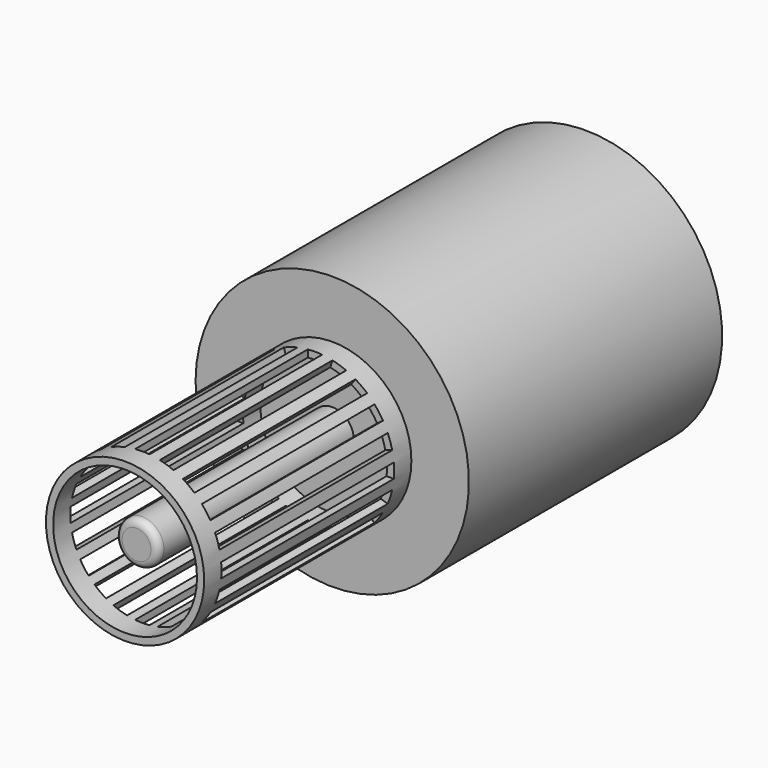
from build123d import *

# Parameters (mm, degrees)
F0_R            = 5.5
F0_R_2          = 5
F1_DEPTH        = 35
F2_W            = 18
F2_H            = 30
F3_DEPTH        = 25
F3_DEPTH_BACK   = 25
F4_R            = 7.5
F4_R_2          = 5.5
F4_R_3          = 5
F5_DEPTH        = 2
F6_W            = 15
F6_H            = 1
F7_DEPTH        = 10
F7_COPIES_COUNT = 20
F8_R            = 1.5
F9_DEPTH        = 19
F11_R           = 9.5
F11_R_2         = 9
F11_R_3         = 7.5
F12_DEPTH       = 2
F13_DEPTH       = 20
F14_R           = 0.5


# Not quite as in the source:
# - a pattern or mirror of a feature is missing from the dataset's text; its kind, count and spacing are read off the source's solid


with BuildPart() as f1:
    # F0 (on Front) → F1 (new body)
    with BuildSketch(Plane.XZ):
        Circle(F0_R)
        Circle(F0_R_2, mode=Mode.SUBTRACT)
    extrude(amount=F1_DEPTH)

    # F2 (on Top) → F3 (cut, two sides)
    with BuildSketch(Plane.XY) as f3_sk:
        Rectangle(F2_W, F2_H)
    extrude(amount=F3_DEPTH, mode=Mode.SUBTRACT)
    extrude(f3_sk.sketch, amount=-F3_DEPTH_BACK, mode=Mode.SUBTRACT)

    # F4 (on face) → F5 (join)
    with BuildSketch(Plane(origin=(0, -15, 0), x_dir=(-1, 0, 0), z_dir=(0, 1, 0))):
        Circle(F4_R)
        Circle(F4_R_2, mode=Mode.SUBTRACT)
        Circle(F4_R_3)
    extrude(amount=-F5_DEPTH)

    # F6 (on Right) → F7 (cut)
    with BuildSketch(Plane.YZ):
        with Locations((-26, 0)):
            Rectangle(F6_W, F6_H)
    f7 = extrude(amount=-F7_DEPTH, mode=Mode.SUBTRACT)

    # F7_copies: F7 ×20 about axis
    f7_copies_axis = Axis((0, 0, 0), (0, 1, 0))
    for i in range(1, F7_COPIES_COUNT):
        add(f7.rotate(f7_copies_axis, i * 360 / F7_COPIES_COUNT), mode=Mode.SUBTRACT)

    # F8 (on face) → F9 (join)
    with BuildSketch(Plane(origin=(0, -15, 0), x_dir=(-1, 0, 0), z_dir=(0, 1, 0))):
        Circle(F8_R)
    extrude(amount=-F9_DEPTH)

    # F11 (on face) → F12 (join)
    with BuildSketch(Plane(origin=(0, -15, 0), x_dir=(-1, 0, 0), z_dir=(0, 1, 0))):
        Circle(F11_R)
        Circle(F11_R_2, mode=Mode.SUBTRACT)
        Circle(F11_R_2)
        Circle(F11_R_3, mode=Mode.SUBTRACT)
    extrude(amount=-F12_DEPTH)

    # F11 (on face) → F13 (join)
    with BuildSketch(Plane(origin=(0, -15, 0), x_dir=(-1, 0, 0), z_dir=(0, 1, 0))):
        Circle(F11_R)
        Circle(F11_R_2, mode=Mode.SUBTRACT)
    extrude(amount=F13_DEPTH)

    # F14
    f14_edges = [f1.edges().sort_by_distance(p)[0] for p in [
        (1.5, -34, 0),
    ]]
    fillet(f14_edges, radius=F14_R)


solid = f1.part
